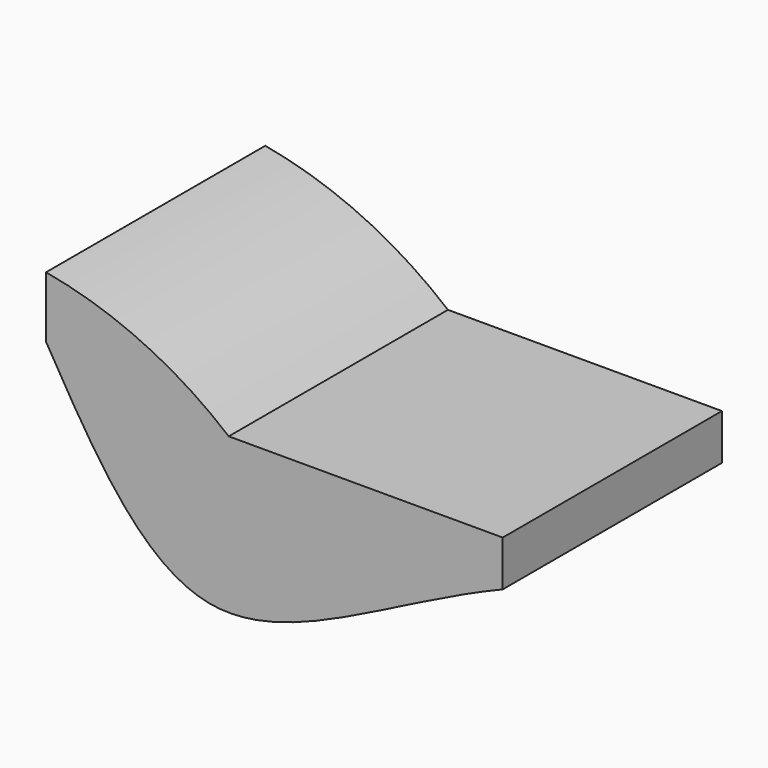
from build123d import *

# Parameters (mm, degrees)
F0_W        = 38.1
F0_H        = 22.86
F1_DEPTH    = 33.02
F4_DEPTH    = 25.4
F5_T1_DEPTH = 128.3541230591


# Not quite as in the source:
# - a fillet or chamfer that OpenCascade refuses, or shapes differently, is made with other operations: its cross-section is extruded or revolved along the edge and cut away or added


with BuildPart() as f1:
    # F0 (on Top) → F1 (new body)
    with BuildSketch(Plane.XY):
        with Locations((19.05, -11.43)):
            Rectangle(F0_W, F0_H)
    extrude(amount=F1_DEPTH)

    # F3 (on face) → F4 (cut)
    with BuildSketch(Plane.XZ.offset(22.86)):
        with BuildLine():
            Line((0, 22.3022773862), (0, 0))
            Line((0, 0), (38.1, 0))
            Line((38.1, 0), (38.1, 16.51))
            add(Edge.make_bspline(
                [(0, 22.3022773862), (4.0173555015, 15.4189654394), (12.5954888388, 0.7212450957), (28.7387394496, 12.7226787633), (38.1, 16.51)],
                knots=[0, 0, 0, 0, 0.2888963968, 0.6168714248, 0.6168714248, 0.6168714248, 0.6168714248], degree=3))
        make_face()
        Polygon((0, 33.02), (0, 27.94), (15.24, 27.94), (15.24, 20.32), (38.1, 20.32), (38.1, 33.02), align=None)
    extrude(amount=-F4_DEPTH, mode=Mode.SUBTRACT)

    # F5: fillet of radius 33.02 on 1 edges, made by hand

    # F5_s2 → F5_t1 (cut)
    with BuildSketch(Plane.XZ.offset(-52.7470615295)):
        with BuildLine():
            ThreePointArc((-5.8588246118, 27.94), (5.3575116884, 25.976628922), (15.24, 20.32))
            Line((15.24, 20.32), (15.24, 27.94))
            Line((15.24, 27.94), (-5.8588246118, 27.94))
        make_face()
    extrude(amount=F5_T1_DEPTH, mode=Mode.SUBTRACT)


solid = f1.part
